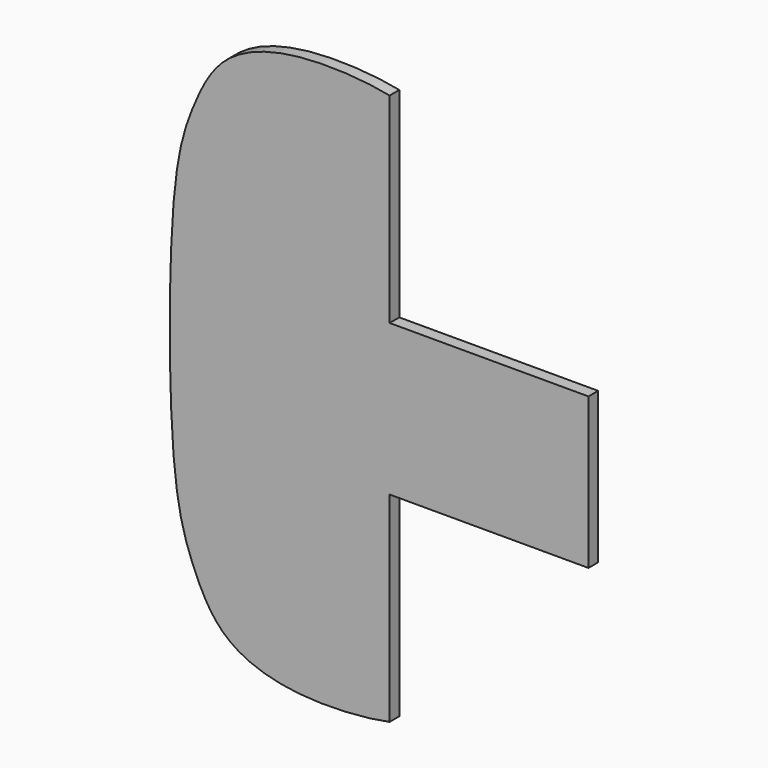
from build123d import *

# Parameters (mm, degrees)
F1_DEPTH = 18


# Not quite as in the source:
# - a feature of the source that left no trace in its solid (it failed there, or was rolled back) is left out


with BuildPart() as f1:
    # F0 (on Front) → F1 (new body)
    with BuildSketch(Plane.XZ):
        with BuildLine():
            Line((295, -217), (-326, -217))
            add(Edge.make_bspline(
                [(0, -626), (-31.9041572511, -632.8686919212), (-135.8624745728, -641.8458876021), (-249.8265846826, -605.2490014373), (-303.9460461433, -495.6098595325), (-325.4699671722, -417.4111427766), (-326, -217)],
                knots=[0, 0, 0, 0, 0.234743673, 0.4538776177, 0.6453771431, 1, 1, 1, 1], degree=3))
            Line((0, -626), (0, -329))
            Line((0, -329), (295, -329))
            Line((295, -329), (295, -217))
        make_face()
        with BuildLine():
            add(Edge.make_bspline(
                [(0, 192), (-31.9041572511, 198.8686919212), (-135.8624745728, 207.8458876021), (-249.8265846826, 171.2490014373), (-303.9460461433, 61.6098595325), (-325.4699671722, -16.5888572234), (-326, -217)],
                knots=[0, 0, 0, 0, 0.234743673, 0.4538776177, 0.6453771431, 1, 1, 1, 1], degree=3))
            Line((-326, -217), (295, -217))
            Line((295, -217), (295, -105))
            Line((295, -105), (0, -105))
            Line((0, -105), (0, 192))
        make_face()
    extrude(amount=F1_DEPTH)


solid = f1.part
